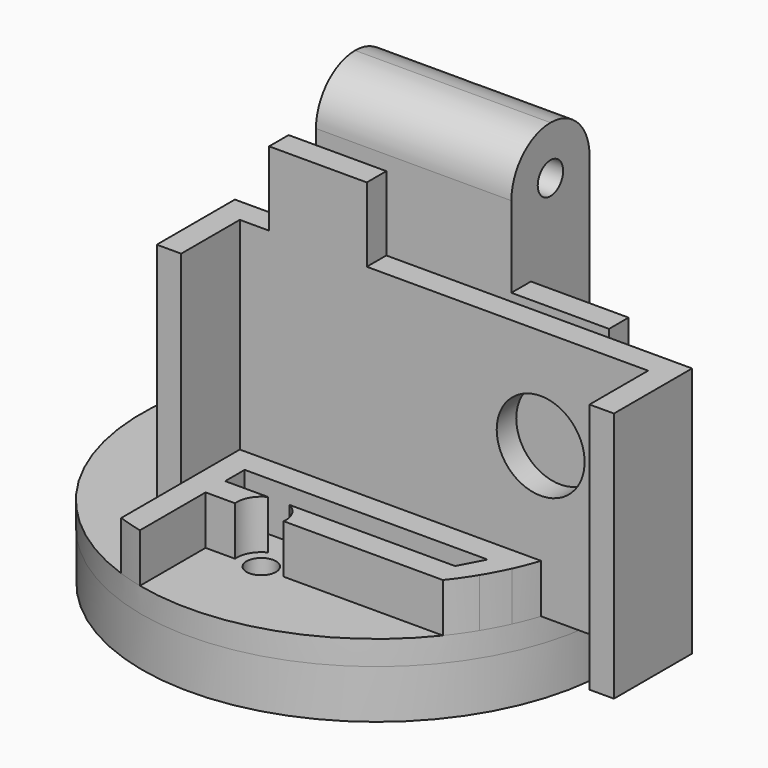
from build123d import *

# Parameters (mm, degrees)
F0_R      = 21.5
F1_DEPTH  = 3
F2_R      = 1.5
F3_DEPTH  = 3
F4_R      = 24
F4_R_2    = 22.25
F5_DEPTH  = 5
F7_R      = 8
F7_R_2    = 7.5
F8_DEPTH  = 3
F6_R      = 24.0393352326
F6_R_2    = 1.5
F9_DEPTH  = 2.5
F10_W     = 41.8
F10_H     = 2.5
F11_DEPTH = 25.7
F12_R     = 4.5
F13_DEPTH = 2.5
F14_W     = 2.5
F14_H     = 2.5
F15_DEPTH = 5
F17_DEPTH = 33.3
F18_R     = 1.625
F19_DEPTH = 20
F20_W     = 10
F20_H     = 2.5
F21_DEPTH = 7.6
F22_W     = 2.5
F22_H     = 5
F23_DEPTH = 5
F24_R     = 1
F25_DEPTH = 2.5
F26_W     = 2.5
F26_H     = 20
F27_DEPTH = 10
F28_R     = 2.5


with BuildPart() as f1:
    # F0 (on Top) → F1 (new body)
    with BuildSketch(Plane.XY):
        Circle(F0_R)
    extrude(amount=F1_DEPTH)

    # F2 (on face) → F3 (cut, through all)
    with BuildSketch(Plane.XY.offset(3)):
        with Locations((0, 14.75)):
            Circle(F2_R)
        with Locations((-14.75, 0)):
            Circle(F2_R)
        with Locations((14.75, 0)):
            Circle(F2_R)
        with Locations((0, -14.75)):
            Circle(F2_R)
    extrude(amount=-F3_DEPTH, mode=Mode.SUBTRACT)

    # F7 (on face) → F8 (join)
    with BuildSketch(Plane(origin=(0, 0, 0), x_dir=(1, 0, 0), z_dir=(0, 0, -1))):
        Circle(F7_R)
        Circle(F7_R_2, mode=Mode.SUBTRACT)
    extrude(amount=F8_DEPTH)


with BuildPart() as f5:
    # F4 (on face) → F5 (new body)
    with BuildSketch(Plane.XY.offset(3)):
        Circle(F4_R)
        Circle(F4_R_2, mode=Mode.SUBTRACT)
    extrude(amount=-F5_DEPTH)

    # F6 (on face) → F9 (join)
    with BuildSketch(Plane.XY.offset(3)):
        Circle(F6_R)
        with Locations((0, -14.75)):
            Circle(F6_R_2, mode=Mode.SUBTRACT)
        with Locations((-14.75, 0)):
            Circle(F6_R_2, mode=Mode.SUBTRACT)
        with Locations((14.75, 0)):
            Circle(F6_R_2, mode=Mode.SUBTRACT)
        with Locations((0, 14.75)):
            Circle(F6_R_2, mode=Mode.SUBTRACT)
    extrude(amount=F9_DEPTH)

    # F10 (on face) → F11 (join)
    with BuildSketch(Plane.XY.offset(5.5)):
        with Locations((12.9, -6.25)):
            Rectangle(F10_W, F10_H)
        Polygon((-8, -7.5), (-8, -5), (-10.5, -5), (-10.5, -15), (-8, -15), align=None)
        Polygon((36.3, -5), (33.8, -5), (33.8, -7.5), (33.8, -15), (36.3, -15), align=None)
    extrude(amount=F11_DEPTH)

    # F12 (on face) → F13 (cut, through all)
    with BuildSketch(Plane(origin=(0, -5, 0), x_dir=(-1, 0, 0), z_dir=(0, 1, 0))):
        with Locations((-22.8, 20.85)):
            Circle(F12_R)
    extrude(amount=-F13_DEPTH, mode=Mode.SUBTRACT)

    # F14 (on face) → F15 (join)
    with BuildSketch(Plane.XY.offset(5.5)):
        with Locations((-6.75, -13.75)):
            Rectangle(F14_W, F14_H)
        Polygon((-8, -7.5), (-8, -12.5), (-5.5, -12.5), (-5.5, -10), (-5.5, -7.5), align=None)
        with BuildLine():
            Line((-5.5, -7.5), (-5.5, -10))
            Line((-5.5, -10), (19.3606870529, -10))
            Line((19.3606870529, -10), (21.8606870529, -10))
            ThreePointArc((21.8606870529, -10), (22.3849872275, -8.7636741867), (22.8394316573, -7.5))
            Line((22.8394316573, -7.5), (-5.5, -7.5))
        make_face()
        with BuildLine():
            Line((21.8606870529, -10), (19.3606870529, -10))
            Line((19.3606870529, -10), (18.0338656474, -12.5))
            Line((18.0338656474, -12.5), (20.5338656474, -12.5))
            ThreePointArc((20.5338656474, -12.5), (21.2341005146, -11.2695436359), (21.8606870529, -10))
        make_face()
        with BuildLine():
            ThreePointArc((2.5, -14.75), (2.4968651828, -14.8751569376), (2.4874685928, -15))
            Line((2.4874685928, -15), (18.7853570215, -15))
            ThreePointArc((18.7853570215, -15), (19.699310085, -13.7777654431), (20.5338656474, -12.5))
            Line((20.5338656474, -12.5), (18.0338656474, -12.5))
            Line((18.0338656474, -12.5), (1.0897247359, -12.5))
            ThreePointArc((1.0897247359, -12.5), (2.1182908015, -13.4222786135), (2.5, -14.75))
        make_face()
        with BuildLine():
            Line((-5.5, -15), (-8, -15))
            Line((-8, -15), (-8, -22.6691340467))
            ThreePointArc((-8, -22.6691340467), (-6.7599307548, -23.0693080654), (-5.5, -23.4017016139))
            Line((-5.5, -23.4017016139), (-5.5, -15))
        make_face()
        with BuildLine():
            Line((-5.5, -12.5), (-5.5, -15))
            Line((-5.5, -15), (-2.4874685928, -15))
            ThreePointArc((-2.4874685928, -15), (-2.1821040369, -13.529990995), (-1.0897247359, -12.5))
            Line((-1.0897247359, -12.5), (-5.5, -12.5))
        make_face()
    extrude(amount=F15_DEPTH)

    # F16 (on face) → F17 (join)
    with BuildSketch(Plane.XY.offset(5.5)):
        with BuildLine():
            Line((-10, 14.75), (-10, 4.75))
            Line((-10, 4.75), (10, 4.75))
            Line((10, 4.75), (10, 14.75))
            Line((10, 14.75), (2.5, 14.75))
            ThreePointArc((2.5, 14.75), (0, 12.25), (-2.5, 14.75))
            Line((-2.5, 14.75), (-10, 14.75))
        make_face()
    extrude(amount=F17_DEPTH)

    # F18 (on face) → F19 (cut, through all)
    with BuildSketch(Plane(origin=(-10, 0, 0), x_dir=(0, -1, 0), z_dir=(-1, 0, 0))):
        with Locations((-9.75, 33.8)):
            Circle(F18_R)
        with BuildLine():
            ThreePointArc((-14.75, 33.8), (-13.2855339059, 37.3355339059), (-9.75, 38.8))
            Line((-9.75, 38.8), (-14.75, 38.8))
            Line((-14.75, 38.8), (-14.75, 33.8))
        make_face()
        with BuildLine():
            ThreePointArc((-9.75, 38.8), (-6.2144660941, 37.3355339059), (-4.75, 33.8))
            Line((-4.75, 33.8), (-4.75, 38.8))
            Line((-4.75, 38.8), (-9.75, 38.8))
        make_face()
    extrude(amount=-F19_DEPTH, mode=Mode.SUBTRACT)

    # F20 (on face) → F21 (join)
    with BuildSketch(Plane.XY.offset(31.2)):
        with Locations((0, -6.25)):
            Rectangle(F20_W, F20_H)
    extrude(amount=F21_DEPTH)

    # F22 (on face) → F23 (join)
    with BuildSketch(Plane.XY.offset(5.5)):
        with Locations((13.75, 8.5)):
            Rectangle(F22_W, F22_H)
    extrude(amount=F23_DEPTH)

    # F24 (on face) → F25 (cut, through all)
    with BuildSketch(Plane.YZ.offset(15)):
        with Locations((8.5, 8)):
            Circle(F24_R)
    extrude(amount=-F25_DEPTH, mode=Mode.SUBTRACT)

    # F26 (on face) → F27 (join)
    with BuildSketch(Plane.YZ.offset(10)):
        with Locations((6, 15.5)):
            Rectangle(F26_W, F26_H)
    extrude(amount=F27_DEPTH)

    # F28
    f28_edges = [f5.edges().sort_by_distance(p)[0] for p in [
        (13.75, 11, 10.5),
    ]]
    fillet(f28_edges, radius=F28_R)


solid = Compound([f1.part, f5.part])
